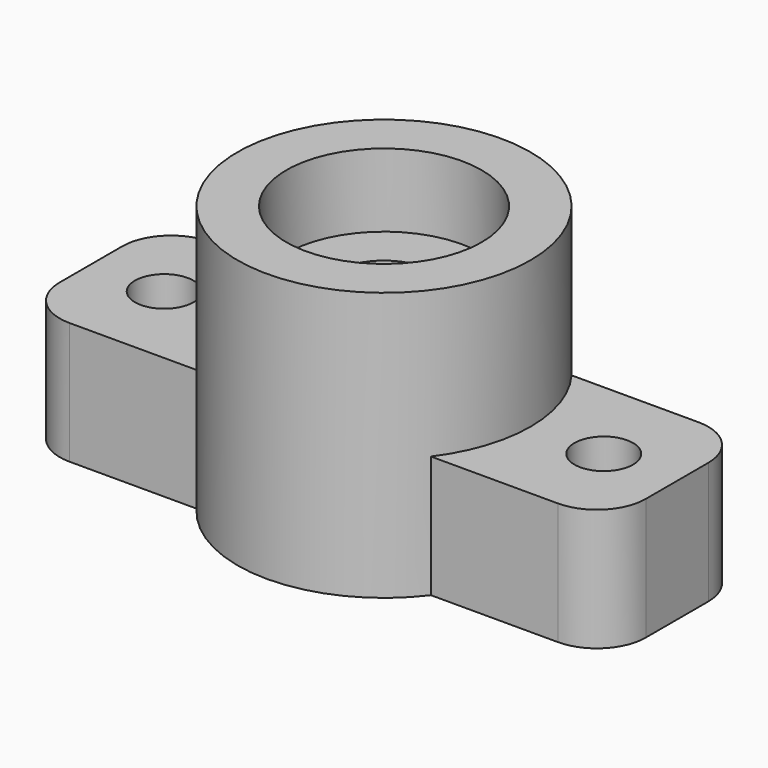
from build123d import *

# Parameters (mm, degrees)
F0_W      = 1200
F0_H      = 360
F1_DEPTH  = 250
F2_R      = 60
F3_DEPTH  = 250.001
F4_R      = 300
F5_DEPTH  = 250.001
F6_R      = 300
F7_DEPTH  = 550
F8_R      = 200
F9_DEPTH  = 150
F10_R     = 100
F11_DEPTH = 400.001
F12_R     = 100


# Not quite as in the source:
# - a feature names something its author has since deleted; it is built from what else it names


with BuildPart() as f1:
    # F0 (on Top) → F1 (new body)
    with BuildSketch(Plane.XY):
        Rectangle(F0_W, F0_H)
    extrude(amount=F1_DEPTH)

    # F2 (on face) → F3 (cut, through all)
    with BuildSketch(Plane.XY.offset(250)):
        with Locations((-450, 0)):
            Circle(F2_R)
        with Locations((450, 0)):
            Circle(F2_R)
    extrude(amount=-F3_DEPTH, mode=Mode.SUBTRACT)

    # F4 (on face) → F5 (cut, through all)
    with BuildSketch(Plane.XY.offset(250)):
        Circle(F4_R)
    extrude(amount=-F5_DEPTH, mode=Mode.SUBTRACT)

    # F6 (on Top) → F7 (join)
    with BuildSketch(Plane.XY):
        Circle(F6_R)
    extrude(amount=F7_DEPTH)

    # F8 (on face) → F9 (cut)
    with BuildSketch(Plane.XY.offset(550)):
        Circle(F8_R)
    extrude(amount=-F9_DEPTH, mode=Mode.SUBTRACT)

    # F10 (on face) → F11 (cut, through all)
    with BuildSketch(Plane.XY.offset(400)):
        Circle(F10_R)
    extrude(amount=-F11_DEPTH, mode=Mode.SUBTRACT)

    # F12
    f12_edges = [f1.edges().sort_by_distance(p)[0] for p in [
        (-600, -180, 125),
        (600, -180, 125),
        (600, 180, 125),
        (-600, 180, 125),
    ]]
    fillet(f12_edges, radius=F12_R)


solid = f1.part
